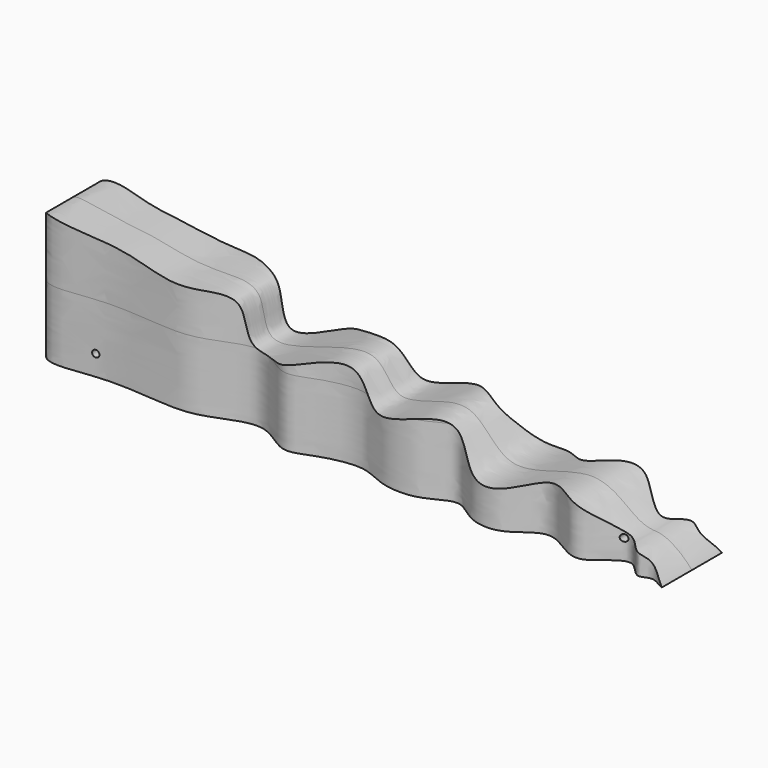
from build123d import *

# Parameters (mm, degrees)
F4_DEPTH = 22.225
F5_DEPTH = 31.75
F6_START = -88.9
F2_R     = 9.525
F6_DEPTH = 63.5
F3_R     = 1.5875
F7_DEPTH = 25.4


with BuildPart() as f4:
    # F0 (on Front) → F4 (new body, symmetric)
    with BuildSketch(Plane.XZ):
        with BuildLine():
            add(Edge.make_bspline(
                [(-145.9356369274, -34.5401912928), (-147.8087758867, -33.1821299753), (-144.4054334454, -20.9567909127), (-145.8003885972, 26.1421511318), (-144.3410158405, 28.0060199983), (-139.7928413345, 28.5675100404), (-121.9316587536, 24.8209943148), (-105.8257803746, 24.0665166702), (-82.268668194, 17.5113324175), (-53.1857759264, 22.4692374088), (-58.1606430321, -12.8129380016), (-0.2981104024, 19.912653563), (4.4457451156, -13.4002981927), (43.0118837466, 11.1397322234), (56.813383113, -25.8583026309), (100.4796968584, 0.6122391617), (118.1357866077, -20.6812033137), (126.9174106938, -21.1611605311), (127.0033571328, -21.1510472108), (134.3912544189, -21.1631162024), (148.0035981402, -34.4655808484), (141.3779205211, -34.5786435746), (121.2203692421, -34.5278027714), (106.2242665559, -34.5438897843), (84.6199133819, -34.5392075337), (65.1618529444, -34.540390496), (53.2295501033, -34.5401228127), (26.5061816728, -34.5401818445), (11.1909749472, -34.5402704062), (-15.2726561901, -34.5397474585), (-49.4888264627, -34.5419233958), (-69.1826648596, -34.5353134901), (-91.8069103323, -34.5581133033), (-107.3884140586, -34.4854449428), (-122.2378775936, -34.7387438713), (-136.4321247579, -33.865771129), (-144.4393800046, -35.6250059765), (-145.9356369274, -34.5401912928)],
                knots=[0, 0, 0, 0, 0.0252833234, 0.0728223462, 0.0813432722, 0.0945759946, 0.1236862119, 0.1520967055, 0.1868759686, 0.2199918001, 0.2489303794, 0.2957258464, 0.3251650614, 0.3636378279, 0.3987916396, 0.4421787325, 0.4761305245, 0.4935351176, 0.4951281527, 0.5128073486, 0.540558091, 0.5522764002, 0.5833260228, 0.611209453, 0.6431785116, 0.673220508, 0.6975974605, 0.7325501076, 0.7601072874, 0.7953737942, 0.8358691227, 0.8669667673, 0.8992845599, 0.926646386, 0.9530633822, 0.9798037687, 1, 1, 1, 1], degree=3))
        make_face()
    extrude(amount=F4_DEPTH, both=True)

    # F1 (on Top) → F5 (intersect, symmetric)
    with BuildSketch(Plane.XY):
        with BuildLine():
            add(Edge.make_bspline(
                [(-146.05, 0), (-146.05, 4.5214745483), (-147.0117106023, 12.2123024311), (-143.6991898837, 17.5820936459), (-134.0214823292, 18.7202317059), (-116.3953285492, 15.1726190971), (-91.5957050288, 17.2934007784), (-72.1387677634, 18.7507065429), (-48.326843793, 4.5647727005), (-32.5852602835, 21.6332248849), (-19.7767953032, 14.9683186069), (0.6359936727, 9.8977027716), (12.8266607352, 18.3849147212), (31.5863878641, 19.2115257672), (44.7378656766, 8.3270699522), (55.4265051461, 20.08800913), (72.2804025491, 21.6121480838), (84.8342439676, 6.9152122355), (98.49389447, 17.016369849), (109.0476505305, 21.0103644902), (123.1805723333, 3.3863020387), (131.2223533637, 18.9476880365), (137.4627593032, 11.6110841385), (149.8462047253, 24.1615356268), (146.05, 4.4612589882), (146.05, 0)],
                knots=[0, 0, 0, 0, 0.0404254681, 0.0664711261, 0.1000419016, 0.1492193585, 0.2066164904, 0.2579890899, 0.314532625, 0.3636429104, 0.4048984458, 0.4561694294, 0.499668618, 0.5481659225, 0.5914916977, 0.6330240544, 0.6781736517, 0.7242674373, 0.7675913812, 0.8044022994, 0.8513245327, 0.8888175099, 0.9175340271, 0.9517675973, 1, 1, 1, 1], degree=3))
            add(Edge.make_bspline(
                [(-146.05, 0), (-146.05, -4.5214745483), (-147.0117106023, -12.2123024311), (-143.6991898837, -17.5820936459), (-134.0214823292, -18.7202317059), (-116.3953285492, -15.1726190971), (-91.5957050288, -17.2934007784), (-72.1387677634, -18.7507065429), (-48.326843793, -4.5647727005), (-32.5852602835, -21.6332248849), (-19.7767953032, -14.9683186069), (0.6359936727, -9.8977027716), (12.8266607352, -18.3849147212), (31.5863878641, -19.2115257672), (44.7378656766, -8.3270699522), (55.4265051461, -20.08800913), (72.2804025491, -21.6121480838), (84.8342439676, -6.9152122355), (98.49389447, -17.016369849), (109.0476505305, -21.0103644902), (123.1805723333, -3.3863020387), (131.2223533637, -18.9476880365), (137.4627593032, -11.6110841385), (149.8462047253, -24.1615356268), (146.05, -4.4612589882), (146.05, 0)],
                knots=[0, 0, 0, 0, 0.0404254681, 0.0664711261, 0.1000419016, 0.1492193585, 0.2066164904, 0.2579890899, 0.314532625, 0.3636429104, 0.4048984458, 0.4561694294, 0.499668618, 0.5481659225, 0.5914916977, 0.6330240544, 0.6781736517, 0.7242674373, 0.7675913812, 0.8044022994, 0.8513245327, 0.8888175099, 0.9175340271, 0.9517675973, 1, 1, 1, 1], degree=3))
        make_face()
    extrude(amount=F5_DEPTH, both=True, mode=Mode.INTERSECT)

    # F2 (on Right) → F6 (cut)
    with BuildSketch(Plane.YZ.offset(F6_START)):
        Circle(F2_R)
    extrude(amount=-F6_DEPTH, mode=Mode.SUBTRACT)

    # F3 (on Front) → F7 (cut, symmetric)
    with BuildSketch(Plane.XZ):
        with Locations((-120.65, -22.225)):
            Circle(F3_R)
        with Locations((120.65, -22.225)):
            Circle(F3_R)
    extrude(amount=F7_DEPTH, both=True, mode=Mode.SUBTRACT)


solid = f4.part
